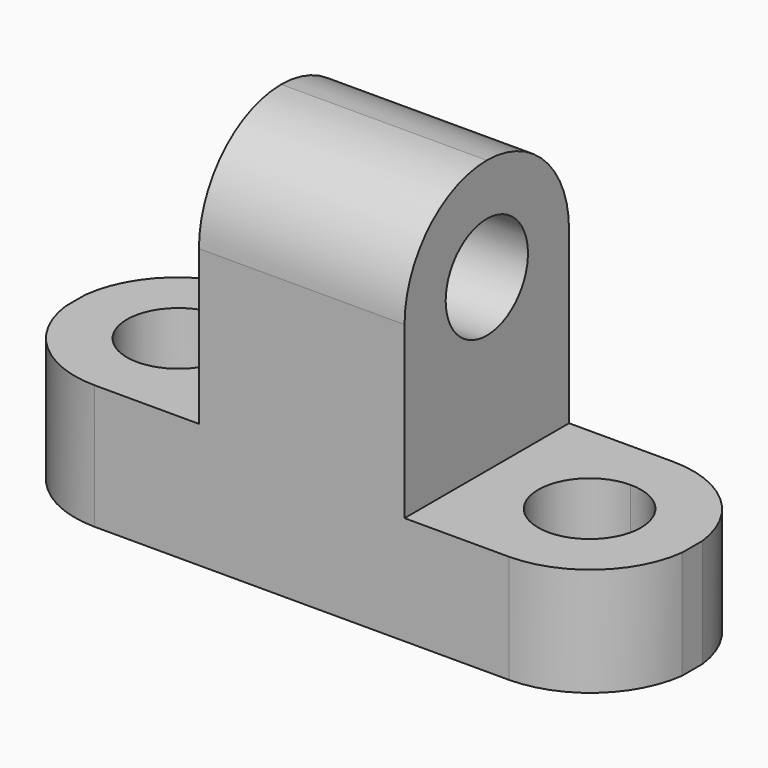
from build123d import *

# Parameters (mm, degrees)
F1_DEPTH = 25.4
F3_DEPTH = 50.801
F5_DEPTH = 13.394231155
F7_DEPTH = 15.3907378061


with BuildPart() as f1:
    # F0 (on Front) → F1 (new body)
    with BuildSketch(Plane.XZ):
        Polygon((-30.3635369193, 15.3897378061), (-30.3635369193, 0), (45.8364630807, 0), (45.8364630807, 13.393231155), (20.4364630807, 13.393231155), (20.4364630807, 47.1397378061), (-4.9635369193, 47.1397378061), (-4.9635369193, 15.3897378061), align=None)
    extrude(amount=F1_DEPTH)

    # F2 (on face) → F3 (cut, through all)
    with BuildSketch(Plane.YZ.offset(20.4364630807)):
        with BuildLine():
            Line((-19.05, 34.4397378061), (-6.35, 34.4397378061))
            ThreePointArc((-6.35, 34.4397378061), (-12.7, 40.7897378061), (-19.05, 34.4397378061))
        make_face()
        with BuildLine():
            ThreePointArc((-25.4, 34.4397378061), (-21.6802561211, 43.4199939272), (-12.7, 47.1397378061))
            Line((-12.7, 47.1397378061), (-25.4, 47.1397378061))
            Line((-25.4, 47.1397378061), (-25.4, 34.4397378061))
        make_face()
        with BuildLine():
            ThreePointArc((-12.7, 47.1397378061), (-3.7197438789, 43.4199939272), (0, 34.4397378061))
            Line((0, 34.4397378061), (0, 47.1397378061))
            Line((0, 47.1397378061), (-12.7, 47.1397378061))
        make_face()
        with BuildLine():
            ThreePointArc((-19.05, 34.4397378061), (-12.7, 28.0897378061), (-6.35, 34.4397378061))
            Line((-6.35, 34.4397378061), (-19.05, 34.4397378061))
        make_face()
    extrude(amount=-F3_DEPTH, mode=Mode.SUBTRACT)

    # F4 (on face) → F5 (cut, through all)
    with BuildSketch(Plane.XY.offset(13.393231155)):
        with BuildLine():
            ThreePointArc((39.4864630807, -12.7), (37.6265911412, -8.2098719395), (33.1364630807, -6.35))
            Line((33.1364630807, -6.35), (33.1364630807, -19.05))
            ThreePointArc((33.1364630807, -19.05), (37.6265911412, -17.1901280605), (39.4864630807, -12.7))
        make_face()
        with BuildLine():
            Line((33.1364630807, -19.05), (33.1364630807, -6.35))
            ThreePointArc((33.1364630807, -6.35), (26.7864630807, -12.7), (33.1364630807, -19.05))
        make_face()
        with BuildLine():
            Line((45.8364630807, 0), (33.33389133, 0))
            ThreePointArc((33.33389133, 0), (41.6741864681, -3.2088005425), (45.8364630807, -11.1165421488))
            Line((45.8364630807, -11.1165421488), (45.8364630807, 0))
        make_face()
        with BuildLine():
            ThreePointArc((45.8364630807, -14.2834578512), (45.9355608404, -12.7), (45.8364630807, -11.1165421488))
            Line((45.8364630807, -11.1165421488), (45.8364630807, -14.2834578512))
        make_face()
        with BuildLine():
            Line((45.8364630807, -25.4), (45.8364630807, -14.2834578512))
            ThreePointArc((45.8364630807, -14.2834578512), (41.6741864681, -22.1911994575), (33.33389133, -25.4))
            Line((33.33389133, -25.4), (45.8364630807, -25.4))
        make_face()
    extrude(amount=-F5_DEPTH, mode=Mode.SUBTRACT)

    # F6 (on face) → F7 (cut, through all)
    with BuildSketch(Plane.XY.offset(15.3897378061)):
        with BuildLine():
            ThreePointArc((-11.3135369193, -12.7), (-13.1734088588, -8.2098719395), (-17.6635369193, -6.35))
            Line((-17.6635369193, -6.35), (-17.6635369193, -19.05))
            ThreePointArc((-17.6635369193, -19.05), (-13.1734088588, -17.1901280605), (-11.3135369193, -12.7))
        make_face()
        with BuildLine():
            Line((-17.6635369193, -19.05), (-17.6635369193, -6.35))
            ThreePointArc((-17.6635369193, -6.35), (-24.0135369193, -12.7), (-17.6635369193, -19.05))
        make_face()
        with BuildLine():
            ThreePointArc((-30.3635369193, -11.1468519042), (-26.2075067106, -3.2177300877), (-17.8534793608, 0))
            Line((-17.8534793608, 0), (-30.3635369193, 0))
            Line((-30.3635369193, 0), (-30.3635369193, -11.1468519042))
        make_face()
        with BuildLine():
            Line((-30.3635369193, -14.2531480958), (-30.3635369193, -11.1468519042))
            ThreePointArc((-30.3635369193, -11.1468519042), (-30.4588632348, -12.7), (-30.3635369193, -14.2531480958))
        make_face()
        with BuildLine():
            ThreePointArc((-17.8534793608, -25.4), (-26.2075067106, -22.1822699123), (-30.3635369193, -14.2531480958))
            Line((-30.3635369193, -14.2531480958), (-30.3635369193, -25.4))
            Line((-30.3635369193, -25.4), (-17.8534793608, -25.4))
        make_face()
    extrude(amount=-F7_DEPTH, mode=Mode.SUBTRACT)


solid = f1.part
